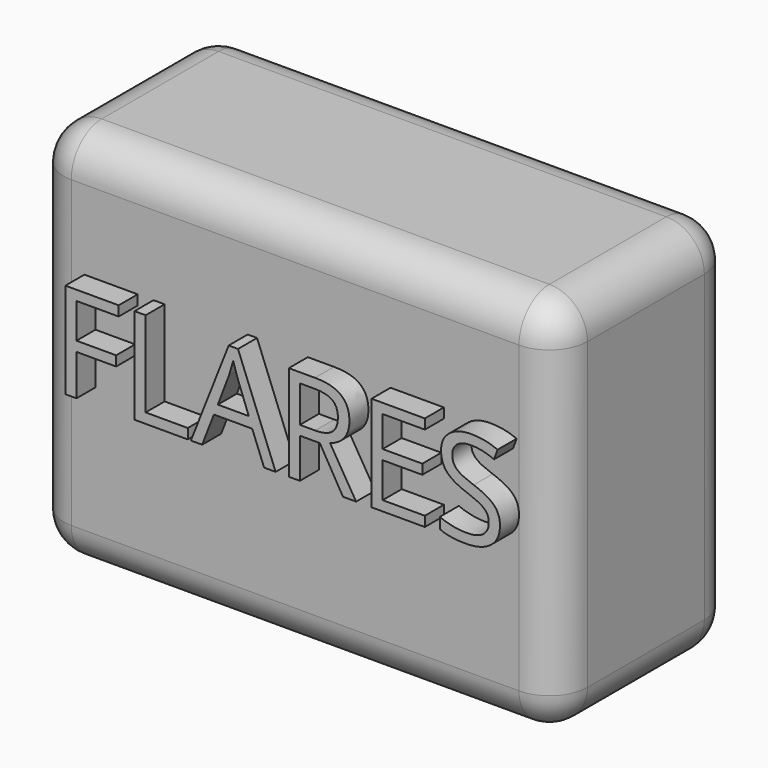
from build123d import *

# Parameters (mm, degrees)
F0_W          = 69.9410811067
F0_H          = 29.6654142439
F1_DEPTH      = 25.4
F1_DEPTH_BACK = 25.4
F2_R          = 5.08
F3_TEXT_SIZE  = 17.8817965546
F4_DEPTH      = 3.175


# Not quite as in the source:
# - a length typed as a fraction of an inch, garbled in the dataset ("3 / 203.2 mm" for 3/8 in), is restored
# - Text() gives the source's letters only with a copy of the font that has no kerning and outlines rounded to 1/6400 em; it was checked with that copy


with BuildPart() as f1:
    # F0 (on Top) → F1 (new body, two sides)
    with BuildSketch(Plane.XY) as f1_sk:
        Rectangle(F0_W, F0_H)
    extrude(amount=F1_DEPTH)
    extrude(f1_sk.sketch, amount=-F1_DEPTH_BACK)

    # F2
    f2_edges = [f1.edges().sort_by_distance(p)[0] for p in [
        (0, 14.832707, 25.4),
        (-34.970541, 14.832707, 0),
        (0, 14.832707, -25.4),
        (34.970541, 14.832707, 0),
        (-34.970541, -14.832707, 0),
        (0, -14.832707, 25.4),
        (34.970541, -14.832707, 0),
        (0, -14.832707, -25.4),
        (34.970541, 0, 25.4),
        (-34.970541, 0, 25.4),
        (-34.970541, 0, -25.4),
        (34.970541, 0, -25.4),
    ]]
    fillet(f2_edges, radius=F2_R)

    # F3 (on face) → F4 (join)
    with BuildSketch(Plane.XZ.offset(14.832707122)):
        with Locations((-29.8905405533, -3.0348771108)):
            Text('FLARES', F3_TEXT_SIZE, font='Open Sans', text_align=(TextAlign.LEFT, TextAlign.BOTTOM))
    extrude(amount=F4_DEPTH)


solid = f1.part
